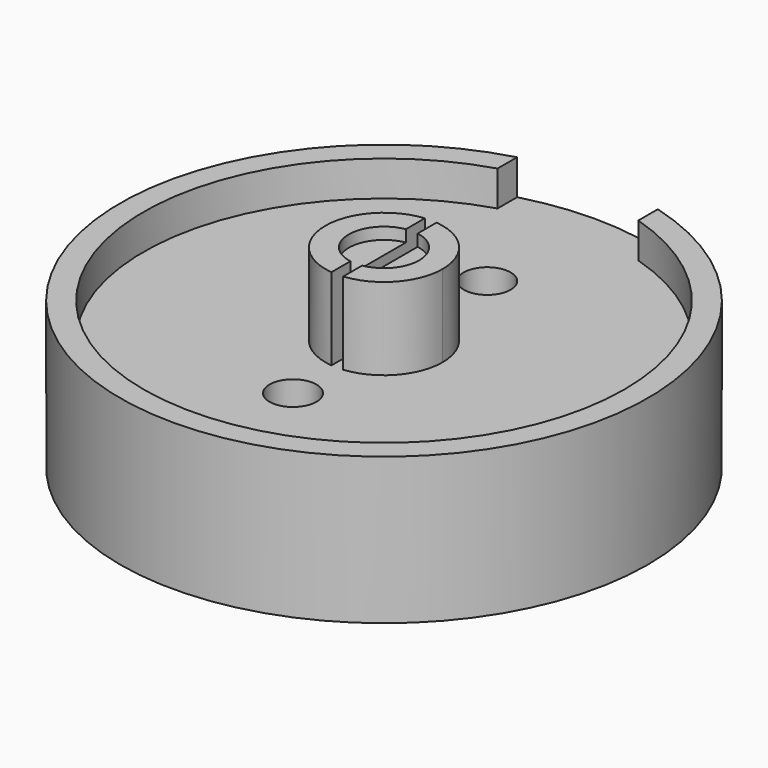
from build123d import *

# Parameters (mm, degrees)
F0_R      = 22.5
F1_DEPTH  = 5.5
F2_R      = 22.5
F2_R_2    = 2
F3_DEPTH  = 4
F5_DEPTH  = 3
F6_DEPTH  = 7
F8_DEPTH  = 1
F10_DEPTH = 1


with BuildPart() as f1:
    # F0 (on Top) → F1 (new body)
    with BuildSketch(Plane.XY):
        Circle(F0_R)
        with BuildLine():
            Line((-3.75, 14), (3.75, 14))
            Line((3.75, 14), (3.75, 8.3714074526))
            ThreePointArc((3.75, 8.3714074526), (9.3641604002, 4.1755149614), (11.5, -2.5))
            ThreePointArc((11.5, -2.5), (-6.6755149614, -11.8641604002), (-3.75, 8.3714074526))
            Line((-3.75, 8.3714074526), (-3.75, 14))
        make_face(mode=Mode.SUBTRACT)
    extrude(amount=F1_DEPTH)

    # F2 (on face) → F3 (join)
    with BuildSketch(Plane.XY.offset(5.5)):
        Circle(F2_R)
        with Locations((0, -9.7)):
            Circle(F2_R_2, mode=Mode.SUBTRACT)
        with Locations((0, 11)):
            Circle(F2_R_2, mode=Mode.SUBTRACT)
    extrude(amount=F3_DEPTH)

    # F4 (on face) → F5 (join)
    with BuildSketch(Plane.XY.offset(9.5)):
        with BuildLine():
            ThreePointArc((-6, 21.6852484422), (-13.6244265934, -17.9060045795), (22.5, 0))
            ThreePointArc((22.5, 0), (17.9060045795, 13.6244265934), (6, 21.6852484422))
            Line((6, 21.6852484422), (6, 19.6022957839))
            ThreePointArc((6, 19.6022957839), (16.4810497238, 12.1911853402), (20.5, 0))
            ThreePointArc((20.5, 0), (-12.1911853402, -16.4810497238), (-6, 19.6022957839))
            Line((-6, 19.6022957839), (-6, 21.6852484422))
        make_face()
    extrude(amount=F5_DEPTH)

    # F4 (on face) → F6 (join)
    with BuildSketch(Plane.XY.offset(9.5)):
        with BuildLine():
            Line((-0.5, -4.9749371855), (-0.5, 4.9749371855))
            ThreePointArc((-0.5, 4.9749371855), (-5, 0), (-0.5, -4.9749371855))
        make_face()
        with BuildLine():
            ThreePointArc((0.5, -4.9749371855), (3.7080992435, -3.3541019662), (5, 0))
            ThreePointArc((5, 0), (3.7080992435, 3.3541019662), (0.5, 4.9749371855))
            Line((0.5, 4.9749371855), (0.5, -4.9749371855))
        make_face()
    extrude(amount=F6_DEPTH)

    # F7 (on face) → F8 (cut)
    with BuildSketch(Plane.XY.offset(16.5)):
        with BuildLine():
            Line((-0.5, -2.9580398915), (-0.5, 2.9580398915))
            ThreePointArc((-0.5, 2.9580398915), (-3, 0), (-0.5, -2.9580398915))
        make_face()
    extrude(amount=-F8_DEPTH, mode=Mode.SUBTRACT)

    # F9 (on face) → F10 (cut)
    with BuildSketch(Plane.XY.offset(16.5)):
        with BuildLine():
            Line((0.5, 2.9580398915), (0.5, -2.9580398915))
            ThreePointArc((0.5, -2.9580398915), (3, 0), (0.5, 2.9580398915))
        make_face()
    extrude(amount=-F10_DEPTH, mode=Mode.SUBTRACT)


solid = f1.part
